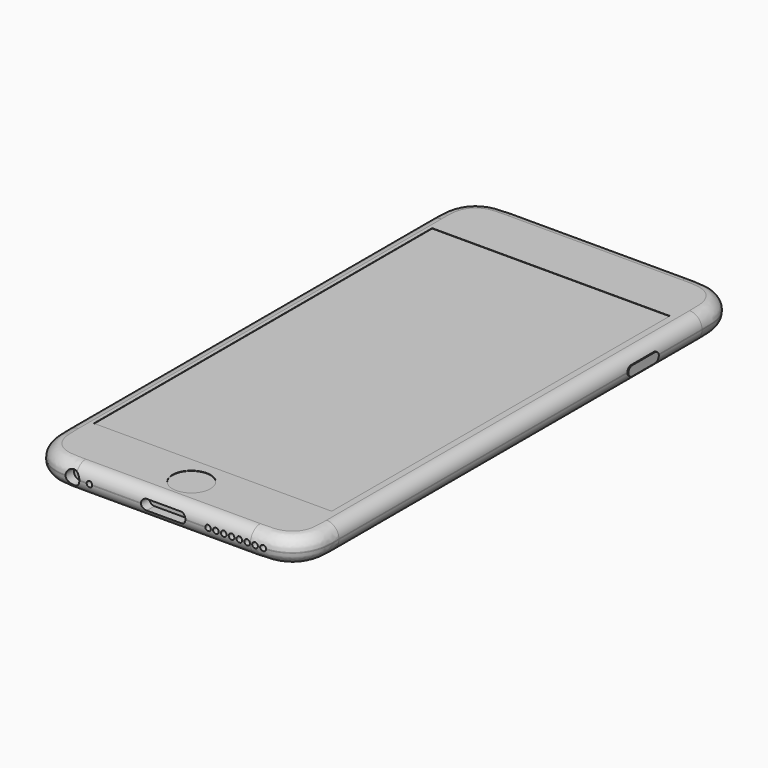
from build123d import *

# Parameters (mm, degrees)
F0_R           = 2.055
F0_R_2         = 0.8
F0_R_3         = 3.83
F1_DEPTH       = 7.3
F2_DEPTH       = 0.67
F3_DEPTH       = 0.1
F4_R           = 5.45
F5_DEPTH       = 0.1
F4_W           = 68.36
F4_H           = 121.54
F6_DEPTH       = 0.1
F10_R          = 3.55
F11_DEPTH      = 3
F11_DEPTH_BACK = 1
F7_R           = 0.8
F13_DEPTH      = 0.3
F14_DEPTH      = 0.3
F15_DEPTH      = 0.43


with BuildPart() as f1:
    # F0 (on Top) → F1 (new body)
    with BuildSketch(Plane.XY):
        with BuildLine():
            Line((-25.09, -79.36), (25.09, -79.36))
            add(Edge.make_bspline(
                [(25.09, -79.36), (25.59, -79.36), (29.3970719372, -79.3863132945), (32.8157812057, -78.6105951637), (36.313364005, -76.453364005), (38.4705951637, -72.9557812057), (39.2463132945, -69.5370719372), (39.22, -65.73), (39.22, -65.23)],
                knots=[0, 0, 0, 0, 0.1670203426, 0.3335413986, 0.5, 0.6664586014, 0.8329796574, 1, 1, 1, 1], degree=3))
            Line((39.22, -65.23), (39.22, 65.23))
            add(Edge.make_bspline(
                [(25.09, 79.36), (25.59, 79.36), (29.3970719372, 79.3863132945), (32.8157812057, 78.6105951637), (36.313364005, 76.453364005), (38.4705951637, 72.9557812057), (39.2463132945, 69.5370719372), (39.22, 65.73), (39.22, 65.23)],
                knots=[0, 0, 0, 0, 0.1670203426, 0.3335413986, 0.5, 0.6664586014, 0.8329796574, 1, 1, 1, 1], degree=3))
            Line((25.09, 79.36), (-25.09, 79.36))
            add(Edge.make_bspline(
                [(-25.09, 79.36), (-25.59, 79.36), (-29.3970719372, 79.3863132945), (-32.8157812057, 78.6105951637), (-36.313364005, 76.453364005), (-38.4705951637, 72.9557812057), (-39.2463132945, 69.5370719372), (-39.22, 65.73), (-39.22, 65.23)],
                knots=[0, 0, 0, 0, 0.1670203426, 0.3335413986, 0.5, 0.6664586014, 0.8329796574, 1, 1, 1, 1], degree=3))
            Line((-39.22, 65.23), (-39.22, -65.23))
            add(Edge.make_bspline(
                [(-25.09, -79.36), (-25.59, -79.36), (-29.3970719372, -79.3863132945), (-32.8157812057, -78.6105951637), (-36.313364005, -76.453364005), (-38.4705951637, -72.9557812057), (-39.2463132945, -69.5370719372), (-39.22, -65.73), (-39.22, -65.23)],
                knots=[0, 0, 0, 0, 0.1670203426, 0.3335413986, 0.5, 0.6664586014, 0.8329796574, 1, 1, 1, 1], degree=3))
        make_face()
        with Locations((13.06, 72.09)):
            Circle(F0_R, mode=Mode.SUBTRACT)
        with Locations((18.16, 72.09)):
            Circle(F0_R_2, mode=Mode.SUBTRACT)
        with Locations((25.12, 72.09)):
            Circle(F0_R_3, mode=Mode.SUBTRACT)
        with Locations((25.12, 72.09)):
            Circle(F0_R_3)
        with Locations((18.16, 72.09)):
            Circle(F0_R_2)
        with Locations((13.06, 72.09)):
            Circle(F0_R)
    extrude(amount=F1_DEPTH)

    # F0 (on Top) → F2 (join)
    with BuildSketch(Plane.XY):
        with Locations((25.12, 72.09)):
            Circle(F0_R_3)
    extrude(amount=-F2_DEPTH)

    # F0 (on Top) → F3 (cut)
    with BuildSketch(Plane.XY):
        with Locations((13.06, 72.09)):
            Circle(F0_R)
        with Locations((18.16, 72.09)):
            Circle(F0_R_2)
    extrude(amount=F3_DEPTH, mode=Mode.SUBTRACT)

    # F4 (on face) → F5 (cut)
    with BuildSketch(Plane.XY.offset(7.3)):
        with Locations((0.32, -69.6)):
            Circle(F4_R)
    extrude(amount=-F5_DEPTH, mode=Mode.SUBTRACT)

    # F4 (on face) → F6 (cut)
    with BuildSketch(Plane.XY.offset(7.3)):
        with Locations((-0.33, -0.33)):
            Rectangle(F4_W, F4_H)
    extrude(amount=-F6_DEPTH, mode=Mode.SUBTRACT)

    # F10
    f10_edges = [f1.edges().sort_by_distance(p)[0] for p in [
        (0, 79.36, 7.3),
        (0, 79.36, 0),
        (0, -79.36, 0),
        (0, -79.36, 7.3),
        (-36.09, -76.23, 0),
        (-36.09, -76.23, 7.3),
        (36.09, -76.23, 0),
        (36.09, -76.23, 7.3),
        (-39.22, 0, 0),
        (39.22, 0, 0),
        (-36.09, 76.23, 0),
        (36.09, 76.23, 0),
        (-39.22, 0, 7.3),
        (39.22, 0, 7.3),
        (-36.09, 76.23, 7.3),
        (36.09, 76.23, 7.3),
    ]]
    fillet(f10_edges, radius=F10_R)


with BuildPart() as f11:
    # F7 (on face) → F11 (new body, two sides)
    with BuildSketch(Plane.XZ.offset(79.36)) as f11_sk:
        with BuildLine():
            Line((-25.09, 1.9064117459), (-25.09, 5.3935882541))
            ThreePointArc((-25.09, 5.3935882541), (-28.1, 3.65), (-25.09, 1.9064117459))
        make_face()
        with BuildLine():
            ThreePointArc((-25.09, 1.9064117459), (-24.350732913, 2.6425031017), (-24.08, 3.65))
            ThreePointArc((-24.08, 3.65), (-24.350732913, 4.6574968983), (-25.09, 5.3935882541))
            Line((-25.09, 5.3935882541), (-25.09, 1.9064117459))
        make_face()
    extrude(amount=-F11_DEPTH)
    extrude(f11_sk.sketch, amount=F11_DEPTH_BACK)


with BuildPart() as f11b:
    # F7 (on face) → F11, piece 2 (new body, two sides)
    with BuildSketch(Plane.XZ.offset(79.36)) as f11_2_sk:
        with Locations((-21.2, 3.65)):
            Circle(F7_R)
    extrude(amount=-F11_DEPTH)
    extrude(f11_2_sk.sketch, amount=F11_DEPTH_BACK)


with BuildPart() as f11c:
    # F7 (on face) → F11, piece 3 (new body, two sides)
    with BuildSketch(Plane.XZ.offset(79.36)) as f11_3_sk:
        with BuildLine():
            Line((4.92, 5.125), (-4.92, 5.125))
            ThreePointArc((-4.92, 5.125), (-6.395, 3.65), (-4.92, 2.175))
            Line((-4.92, 2.175), (4.92, 2.175))
            ThreePointArc((4.92, 2.175), (5.9629825023, 2.6070174977), (6.395, 3.65))
            ThreePointArc((6.395, 3.65), (5.9629825023, 4.6929825023), (4.92, 5.125))
        make_face()
    extrude(amount=-F11_DEPTH)
    extrude(f11_3_sk.sketch, amount=F11_DEPTH_BACK)


with BuildPart() as f11d:
    # F7 (on face) → F11, piece 4 (new body, two sides)
    with BuildSketch(Plane.XZ.offset(79.36)) as f11_4_sk:
        with Locations((12.9, 3.65)):
            Circle(F7_R)
    extrude(amount=-F11_DEPTH)
    extrude(f11_4_sk.sketch, amount=F11_DEPTH_BACK)


with BuildPart() as f11e:
    # F7 (on face) → F11, piece 5 (new body, two sides)
    with BuildSketch(Plane.XZ.offset(79.36)) as f11_5_sk:
        with Locations((15.15, 3.65)):
            Circle(F7_R)
    extrude(amount=-F11_DEPTH)
    extrude(f11_5_sk.sketch, amount=F11_DEPTH_BACK)


with BuildPart() as f11f:
    # F7 (on face) → F11, piece 6 (new body, two sides)
    with BuildSketch(Plane.XZ.offset(79.36)) as f11_6_sk:
        with Locations((17.4, 3.65)):
            Circle(F7_R)
    extrude(amount=-F11_DEPTH)
    extrude(f11_6_sk.sketch, amount=F11_DEPTH_BACK)


with BuildPart() as f11g:
    # F7 (on face) → F11, piece 7 (new body, two sides)
    with BuildSketch(Plane.XZ.offset(79.36)) as f11_7_sk:
        with Locations((19.65, 3.65)):
            Circle(F7_R)
    extrude(amount=-F11_DEPTH)
    extrude(f11_7_sk.sketch, amount=F11_DEPTH_BACK)


with BuildPart() as f11h:
    # F7 (on face) → F11, piece 8 (new body, two sides)
    with BuildSketch(Plane.XZ.offset(79.36)) as f11_8_sk:
        with Locations((21.9, 3.65)):
            Circle(F7_R)
    extrude(amount=-F11_DEPTH)
    extrude(f11_8_sk.sketch, amount=F11_DEPTH_BACK)


with BuildPart() as f11i:
    # F7 (on face) → F11, piece 9 (new body, two sides)
    with BuildSketch(Plane.XZ.offset(79.36)) as f11_9_sk:
        with Locations((24.15, 3.65)):
            Circle(F7_R)
    extrude(amount=-F11_DEPTH)
    extrude(f11_9_sk.sketch, amount=F11_DEPTH_BACK)


with BuildPart() as f11j:
    # F7 (on face) → F11, piece 10 (new body, two sides)
    with BuildSketch(Plane.XZ.offset(79.36)) as f11_10_sk:
        with Locations((26.4, 3.65)):
            Circle(F7_R)
    extrude(amount=-F11_DEPTH)
    extrude(f11_10_sk.sketch, amount=F11_DEPTH_BACK)


with BuildPart() as f11k:
    # F7 (on face) → F11, piece 11 (new body, two sides)
    with BuildSketch(Plane.XZ.offset(79.36)) as f11_11_sk:
        with Locations((28.65, 3.65)):
            Circle(F7_R)
    extrude(amount=-F11_DEPTH)
    extrude(f11_11_sk.sketch, amount=F11_DEPTH_BACK)


with BuildPart() as f1_1:
    add(f1.part)

    # F12: cut F11, F11b, F11d, F11e, F11f, F11g, F11h, F11i, F11j, F11k, F11c
    add(f11.part, mode=Mode.SUBTRACT)
    add(f11b.part, mode=Mode.SUBTRACT)
    add(f11d.part, mode=Mode.SUBTRACT)
    add(f11e.part, mode=Mode.SUBTRACT)
    add(f11f.part, mode=Mode.SUBTRACT)
    add(f11g.part, mode=Mode.SUBTRACT)
    add(f11h.part, mode=Mode.SUBTRACT)
    add(f11i.part, mode=Mode.SUBTRACT)
    add(f11j.part, mode=Mode.SUBTRACT)
    add(f11k.part, mode=Mode.SUBTRACT)
    add(f11c.part, mode=Mode.SUBTRACT)

    # F8 (on face) → F13 (join)
    with BuildSketch(Plane.YZ.offset(39.22)):
        with BuildLine():
            ThreePointArc((39.81, 5.05), (38.41, 3.65), (39.81, 2.25))
            Line((39.81, 2.25), (47.95, 2.25))
            ThreePointArc((47.95, 2.25), (49.35, 3.65), (47.95, 5.05))
            Line((47.95, 5.05), (39.81, 5.05))
        make_face()
    extrude(amount=F13_DEPTH)

    # F9 (on face) → F14 (join)
    with BuildSketch(Plane(origin=(-39.22, 0, 0), x_dir=(0, -1, 0), z_dir=(-1, 0, 0))):
        with BuildLine():
            ThreePointArc((-35.27, 5.03), (-36.67, 3.63), (-35.27, 2.23))
            Line((-35.27, 2.23), (-27.13, 2.23))
            ThreePointArc((-27.13, 2.23), (-25.73, 3.63), (-27.13, 5.03))
            Line((-27.13, 5.03), (-35.27, 5.03))
        make_face()
        with BuildLine():
            ThreePointArc((-47.88, 5.03), (-49.28, 3.63), (-47.88, 2.23))
            Line((-47.88, 2.23), (-39.74, 2.23))
            ThreePointArc((-39.74, 2.23), (-38.34, 3.63), (-39.74, 5.03))
            Line((-39.74, 5.03), (-47.88, 5.03))
        make_face()
    extrude(amount=F14_DEPTH)

    # F9 (on face) → F15 (join)
    with BuildSketch(Plane(origin=(-39.22, 0, 0), x_dir=(0, -1, 0), z_dir=(-1, 0, 0))):
        with BuildLine():
            ThreePointArc((-59.595, 4.63), (-60.58, 3.645), (-59.595, 2.66))
            Line((-59.595, 2.66), (-55.955, 2.66))
            ThreePointArc((-55.955, 2.66), (-54.97, 3.645), (-55.955, 4.63))
            Line((-55.955, 4.63), (-59.595, 4.63))
        make_face()
    extrude(amount=F15_DEPTH)


solid = f1_1.part
